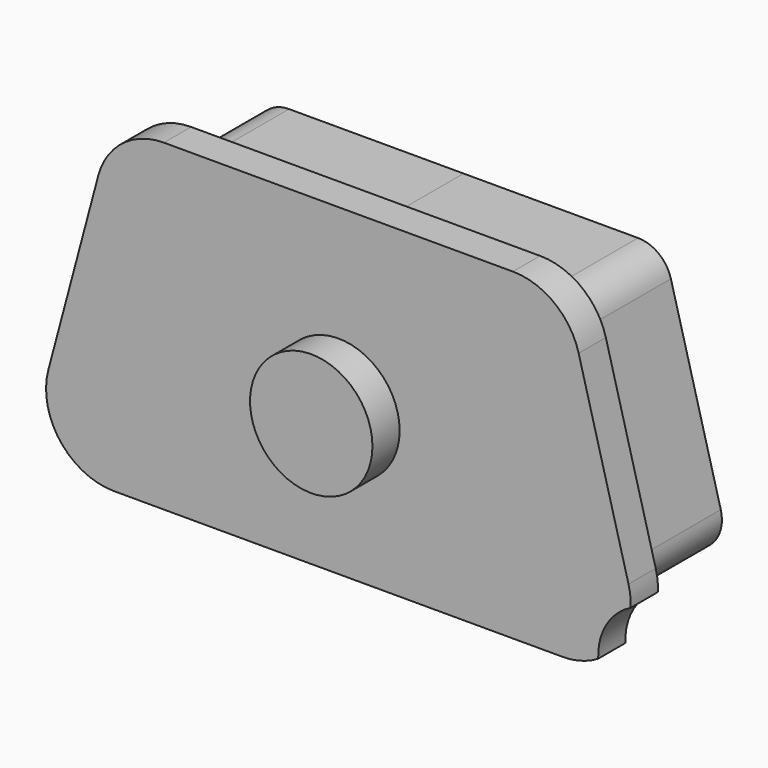
from build123d import *

# Parameters (mm, degrees)
F1_DEPTH = 3.6
F2_W     = 2
F2_H     = 9.5
F3_DEPTH = 1
F4_R     = 1.7401329742
F5_DEPTH = 25
F6_R     = 1.8
F7_DEPTH = 1


# Not quite as in the source:
# - a pattern or mirror of a feature is missing from the dataset's text; its kind, count and spacing are read off the source's solid
# - a feature names something its author has since deleted; it is built from what else it names


with BuildPart() as f1:
    # F0 (on Front) → F1 (new body)
    with BuildSketch(Plane.XZ):
        with BuildLine():
            Line((0, 7.5), (0, 0))
            Line((0, 0), (6.5983883536, 0))
            ThreePointArc((6.5983883536, 0), (7.3913772093, 0.3907638596), (7.5646232932, 1.2576626506))
            Line((7.5646232932, 1.2576626506), (6.0979566265, 6.7576626506))
            ThreePointArc((6.0979566265, 6.7576626506), (5.7409578273, 7.2929888557), (5.1317216869, 7.5))
            Line((5.1317216869, 7.5), (0, 7.5))
        make_face()
    extrude(amount=F1_DEPTH)


with BuildPart() as f1_copies_1:
    # F1_copies: instance of F1
    add(f1.part.mirror(Plane(origin=(0, 0, 0), x_dir=(0, 0, -1), z_dir=(-1, 0, 0))))


with BuildPart() as f3:
    # F2 (on face) → F3 (new body)
    with BuildSketch(Plane.XZ.offset(3.6)):
        with BuildLine():
            Line((1, -1), (6.5983883536, -1))
            ThreePointArc((6.5983883536, -1), (8.184366065, -0.2184722807), (8.5308582328, 1.5153253011))
            Line((8.5308582328, 1.5153253011), (7.0641915661, 7.0153253011))
            ThreePointArc((7.0641915661, 7.0153253011), (6.3501939676, 8.0859777114), (5.1317216869, 8.5))
            Line((5.1317216869, 8.5), (1, 8.5))
            Line((1, 8.5), (1, -1))
        make_face()
        with Locations((0, 3.75)):
            Rectangle(F2_W, F2_H)
        with BuildLine():
            Line((-6.5983883536, -1), (-1, -1))
            Line((-1, -1), (-1, 8.5))
            Line((-1, 8.5), (-5.1317216869, 8.5))
            ThreePointArc((-5.1317216869, 8.5), (-6.3501939676, 8.0859777114), (-7.0641915661, 7.0153253011))
            Line((-7.0641915661, 7.0153253011), (-8.5308582328, 1.5153253011))
            ThreePointArc((-8.5308582328, 1.5153253011), (-8.184366065, -0.2184722807), (-6.5983883536, -1))
        make_face()
    extrude(amount=F3_DEPTH)

    # F4 (on face) → F5 (cut)
    with BuildSketch(Plane(origin=(0, -3.6, 0), x_dir=(-1, 0, 0), z_dir=(0, 1, 0))):
        with Locations((-9.3786362559, -0.6318259402)):
            Circle(F4_R)
    extrude(amount=-F5_DEPTH, mode=Mode.SUBTRACT)

    # F6 (on face) → F7 (join)
    with BuildSketch(Plane.XZ.offset(4.6)):
        with Locations((0, 3.3)):
            Circle(F6_R)
    extrude(amount=F7_DEPTH)


solid = Compound([f1.part, f1_copies_1.part, f3.part])
